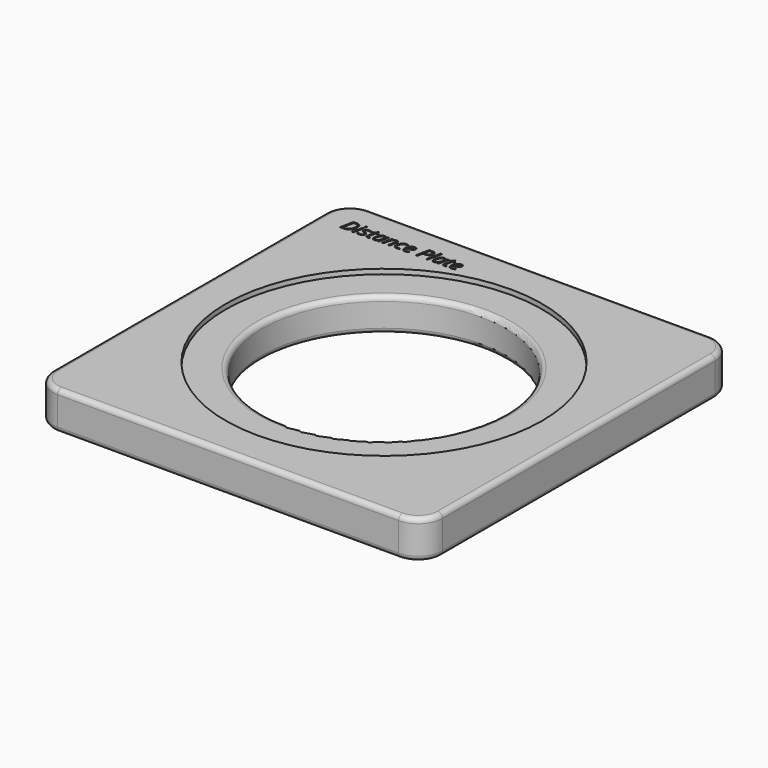
from build123d import *

# Parameters (mm, degrees)
F0_W         = 80
F0_H         = 80
F1_DEPTH     = 3.925
F2_R         = 32.5
F3_DEPTH     = 1
F4_R         = 25
F5_DEPTH     = 25
F6_R         = 5
F7_R         = 1
F8_TEXT_SIZE = 3.8781976277
F9_DEPTH     = 0.5


# Not quite as in the source:
# - Text() gives the source's letters only with a copy of the font that has no kerning and outlines rounded to 1/6400 em; it was checked with that copy


with BuildPart() as f1:
    # F0 (on Top) → F1 (new body, symmetric)
    with BuildSketch(Plane.XY):
        with Locations((-1.8626e-06, 0)):
            Rectangle(F0_W, F0_H)
    extrude(amount=F1_DEPTH, both=True)

    # F2 (on face) → F3 (cut)
    with BuildSketch(Plane.XY.offset(3.925)):
        Circle(F2_R)
    extrude(amount=-F3_DEPTH, mode=Mode.SUBTRACT)

    # F4 (on face) → F5 (cut)
    with BuildSketch(Plane.XY.offset(2.925)):
        Circle(F4_R)
    extrude(amount=-F5_DEPTH, mode=Mode.SUBTRACT)

    # F6
    f6_edges = [f1.edges().sort_by_distance(p)[0] for p in [
        (39.999998, -40, 0),
        (39.999998, 40, 0),
        (-40.000002, -40, 0),
        (-40.000002, 40, 0),
    ]]
    fillet(f6_edges, radius=F6_R)

    # F7
    f7_edges = [f1.edges().sort_by_distance(p)[0] for p in [
        (-2e-06, 40, 3.925),
        (-25, 0, 2.925),
        (-25, 0, -3.925),
        (-2e-06, -40, -3.925),
    ]]
    fillet(f7_edges, radius=F7_R)

    # F8 (on face) → F9 (cut)
    with BuildSketch(Plane.XY.offset(3.925)):
        with Locations((-35.0000018626, 32.2076977081)):
            Text('Distance Plate', F8_TEXT_SIZE, font='Open Sans', font_style=FontStyle.ITALIC, text_align=(TextAlign.LEFT, TextAlign.BOTTOM))
    extrude(amount=-F9_DEPTH, mode=Mode.SUBTRACT)


solid = f1.part
